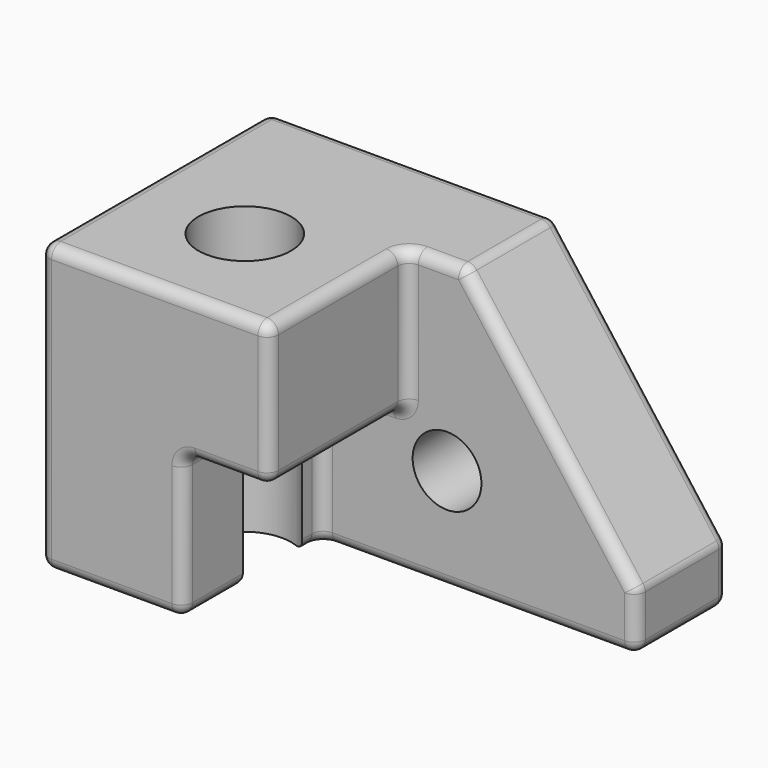
from build123d import *

# Parameters (mm, degrees)
F0_W     = 203.2
F0_H     = 127
F1_DEPTH = 127
F3_DEPTH = 76.2
F4_SIZE2 = 101.6
F4_SIZE  = 76.2
F5_R     = 5.08
F6_R     = 15.24
F7_DEPTH = 50.8
F8_R     = 20.5391892085
F9_DEPTH = 127


with BuildPart() as f1:
    # F0 (on Front) → F1 (new body)
    with BuildSketch(Plane.XZ):
        with Locations((2.9485966027, -0.464142194)):
            Rectangle(F0_W, F0_H)
    extrude(amount=F1_DEPTH)

    # F2 (on face) → F3 (cut)
    with BuildSketch(Plane.XZ.offset(127)):
        Polygon((-35.1514033973, 0), (-35.1514033973, -63.964142194), (104.5485966027, -63.964142194), (104.5485966027, 63.035857806), (2.9485966027, 63.035857806), (2.9485966027, 0), align=None)
    extrude(amount=-F3_DEPTH, mode=Mode.SUBTRACT)

    # F4
    f4_edges = [f1.edges().sort_by_distance(p)[0] for p in [
        (104.548597, -25.4, 63.035858),
    ]]
    f4_side = f1.faces().sort_by_distance((-18.822832, -52.614286, 63.035858))[0]
    chamfer(f4_edges, length=F4_SIZE, length2=F4_SIZE2, reference=f4_side)

    # F5
    f5_edges = [f1.edges().sort_by_distance(p)[0] for p in [
        (-98.651403, -63.5, 63.035858),
        (-47.851403, -127, 63.035858),
        (2.948597, -88.9, 63.035858),
        (15.648597, -50.8, 63.035858),
        (28.348597, -25.4, 63.035858),
        (-35.151403, 0, 63.035858),
        (2.948597, -127, 31.517929),
        (2.948597, -88.9, 0),
        (-35.151403, -127, -31.982071),
        (-16.101403, -127, 0),
        (-16.101403, -50.8, 0),
        (-35.151403, -88.9, 0),
        (-35.151403, -50.8, -31.982071),
        (-66.901403, -127, -63.964142),
        (-35.151403, -88.9, -63.964142),
        (34.698597, -50.8, -63.964142),
        (104.548597, -25.4, -63.964142),
        (104.548597, -50.8, -51.264142),
        (104.548597, 0, -51.264142),
        (104.548597, -25.4, -38.564142),
        (66.448597, 0, 12.235858),
        (66.448597, -50.8, 12.235858),
        (-98.651403, 0, -0.464142),
        (2.948597, 0, -63.964142),
        (-98.651403, -63.5, -63.964142),
        (-98.651403, -127, -0.464142),
        (2.948597, -50.8, 31.517929),
    ]]
    fillet(f5_edges, radius=F5_R)

    # F6 (on face) → F7 (cut, through all)
    with BuildSketch(Plane.XZ.offset(50.8)):
        with Locations((20.7285966027, -18.244142194)):
            Circle(F6_R)
    extrude(amount=-F7_DEPTH, mode=Mode.SUBTRACT)

    # F8 (on face) → F9 (cut, through all)
    with BuildSketch(Plane.XY.offset(63.035857806)):
        with Locations((-47.4430248141, -77.6382982731)):
            Circle(F8_R)
    extrude(amount=-F9_DEPTH, mode=Mode.SUBTRACT)


solid = f1.part
